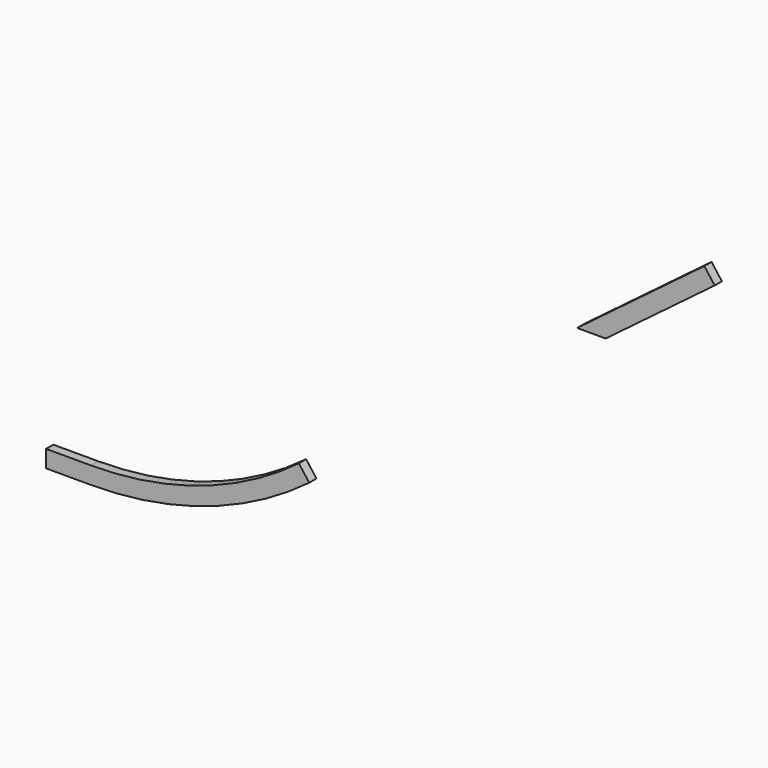
from build123d import *

# Parameters (mm, degrees)
F1_DEPTH = 10


# Not quite as in the source:
# - a feature names something its author has since deleted; it is built from what else it names


with BuildPart() as f1:
    # F0 (on Front) → F1 (new body)
    with BuildSketch(Plane.XZ):
        with BuildLine():
            Line((-136.214891398, -230.3754368354), (-147.6493768378, -215.2013621445))
            ThreePointArc((-147.6493768378, -215.2013621445), (-256.0478265684, -272.23254545), (-376.9409006588, -291.9212328165))
            Line((-376.9409006588, -291.9212328165), (-426.9409006588, -291.9212328165))
            Line((-426.9409006588, -291.9212328165), (-426.9409006588, -310.9212328165))
            Line((-426.9409006588, -310.9212328165), (-376.9409006588, -310.9212328165))
            ThreePointArc((-376.9409006588, -310.9212328165), (-250.0190380967, -290.250694899), (-136.214891398, -230.3754368354))
        make_face()
    extrude(amount=F1_DEPTH)


with BuildPart() as f1b:
    # F0 (on Front) → F1, piece 2 (new body)
    with BuildSketch(Plane.XZ):
        Polygon((311.7478876598, 107.1887296189), (300.3134022199, 122.3628043098), (159.7403426108, 16.433405906), (191.3115052921, 16.433405906), align=None)
    extrude(amount=F1_DEPTH)


solid = Compound([f1.part, f1b.part])
